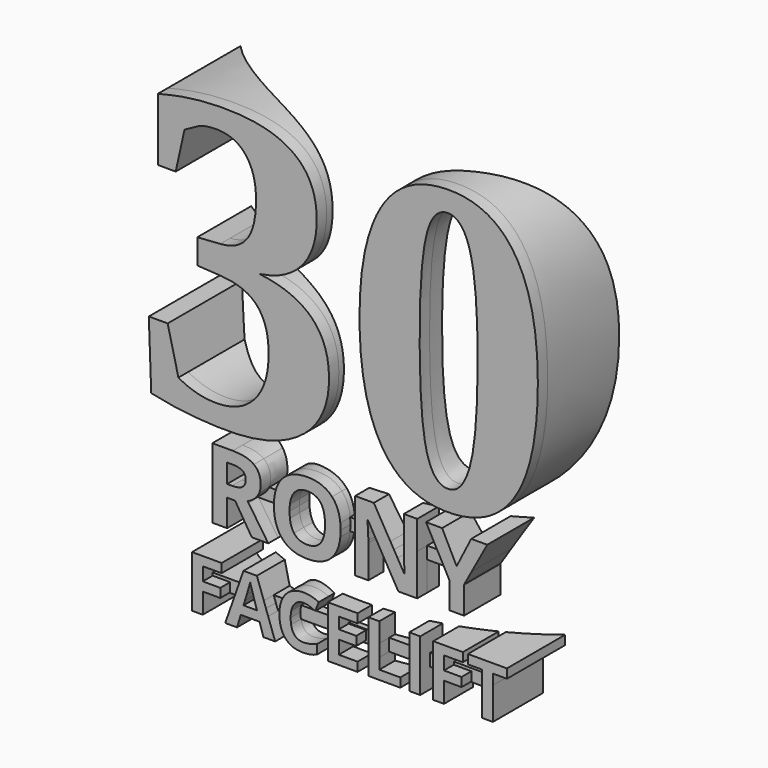
from build123d import *

# Parameters (mm, degrees)
F0_TEXT_SIZE = 68.3343502135
F0_W         = 2.1540381229
F0_H         = 4.7308358373
F0_W_2       = 2.1689621745
F0_H_2       = 4.6338295015
F0_W_3       = 1.7499570325
F0_H_3       = 3.2307460681
F0_W_4       = 1.7793372135
F0_H_4       = 3.1591318768
F0_W_5       = 4.8605836989
F0_H_5       = 1
F0_W_6       = 2.1117005114
F1_DEPTH     = 30
F2_R         = 41.5
F3_DEPTH     = 100
F5_DEPTH     = 2


# Not quite as in the source:
# - Text() gives the source's letters only with a copy of the font that has no kerning and outlines rounded to 1/6400 em; it was checked with that copy


with BuildPart() as f1:
    # F0 (on Front) → F1 (new body)
    with BuildSketch(Plane.XZ):
        with Locations((-35, 14.6143996297)):
            Text('30', F0_TEXT_SIZE, font='Tinos', font_style=FontStyle.BOLD, text_align=(TextAlign.LEFT, TextAlign.BOTTOM))
        with BuildLine():
            Line((-16.2295685047, 4.7308358373), (-22.1137135467, 4.7308358373))
            Line((-22.1137135467, 4.7308358373), (-22.1137135467, 0))
            Line((-22.1137135467, 0), (-19.7034792037, 0))
            Line((-19.7034792037, 0), (-19.7034792037, 4.3603104266))
            Line((-19.7034792037, 4.3603104266), (-18.4224981029, 4.3603104266))
            Line((-18.4224981029, 4.3603104266), (-15.7088080428, 0))
            Line((-15.7088080428, 0), (-13.0349154537, 0))
            add(Edge.make_bspline(
                [(-16.2295685047, 4.7308358373), (-13.7883128068, 1.0866307977), (-13.0349154537, 0)],
                knots=[0.0291905331, 0.0291905331, 0.0291905331, 1, 1, 1], degree=2))
        make_face()
        with Locations((2.1428450841, 2.3654179187)):
            Rectangle(F0_W, F0_H)
        with Locations((10.0625418315, 9.0477505881)):
            Rectangle(F0_W_2, F0_H_2)
        Polygon((17.5671948611, 6.7308358373), (17.521881029, 6.7308358373), (17.5444663969, 6.6859751435), align=None)
        Polygon((17.5671948611, 6.7308358373), (19.994710284, 6.7308358373), (22.5116882576, 11.3646653388), (19.9149032689, 11.3646653388), align=None)
        Polygon((18.9083613052, 4.7308358373), (16.1409885207, 4.7308358373), (16.3480549222, 4.3453863749), (16.3480549222, 0), (18.7408778716, 0), (18.7408778716, 4.4224939751), align=None)
        Polygon((12.5772445362, 11.3646653388), (15.0665732124, 6.7308358373), (17.521881029, 6.7308358373), (15.1889535766, 11.3646653388), align=None)
        with Locations((-24.5407143345, -12.0396394394)):
            Rectangle(F0_W_3, F0_H_3)
        Polygon((-25.4156928507, -5.2651345286), (-25.4156928507, -8.4242664054), (-23.6657358182, -8.4242664054), (-23.6657358182, -6.7231260121), (-20.6065244687, -6.7231260121), (-20.6065244687, -5.2651345286), align=None)
        Polygon((-13.051883354, -10.4242664054), (-18.8849259394, -10.4242664054), (-20.0207571094, -13.6550124735), (-18.1037002973, -13.6550124735), (-17.4958978023, -11.6571601635), (-14.4366864527, -11.6571601635), (-13.8288839577, -13.6550124735), (-11.9118271456, -13.6550124735), align=None)
        with BuildLine():
            add(Edge.make_bspline(
                [(-11.143774011, -8.4242664054), (-11.0275262467, -7.7471500045), (-10.7522281257, -7.1785188181)],
                knots=[0.4222613792, 0.4222613792, 0.4222613792, 1, 1, 1], degree=2))
            Line((-11.143774011, -8.4242664054), (-9.2940985776, -8.4242664054))
            add(Edge.make_bspline(
                [(-8.8471070121, -7.3805075626), (-9.158759552, -7.8074715422), (-9.2940985776, -8.4242664054)],
                knots=[0, 0, 0, 0.5657374533, 0.5657374533, 0.5657374533], degree=2))
            add(Edge.make_bspline(
                [(-7.2917936789, -6.6258041625), (-8.2962286178, -6.6258041625), (-8.8471070121, -7.3805075626)],
                knots=[0, 0, 0, 1, 1, 1], degree=2))
            add(Edge.make_bspline(
                [(-6.35713667, -6.7919858114), (-6.8327283504, -6.6258041625), (-7.2917936789, -6.6258041625)],
                knots=[0, 0, 0, 1, 1, 1], degree=2))
            add(Edge.make_bspline(
                [(-5.4096258318, -7.1821913407), (-5.8815449896, -6.9581674603), (-6.35713667, -6.7919858114)],
                knots=[0, 0, 0, 1, 1, 1], degree=2))
            Line((-5.4096258318, -7.1821913407), (-4.8367123018, -5.7352174251))
            add(Edge.make_bspline(
                [(-7.2917936789, -5.1457775432), (-6.070679905, -5.1457775432), (-4.8367123018, -5.7352174251)],
                knots=[0, 0, 0, 1, 1, 1], degree=2))
            add(Edge.make_bspline(
                [(-9.3832953159, -5.6700301484), (-8.4908723171, -5.1457775432), (-7.2917936789, -5.1457775432)],
                knots=[0, 0, 0, 1, 1, 1], degree=2))
            add(Edge.make_bspline(
                [(-10.7522281257, -7.1785188181), (-10.2757183146, -6.1942827536), (-9.3832953159, -5.6700301484)],
                knots=[0, 0, 0, 1, 1, 1], degree=2))
        make_face()
        with BuildLine():
            Line((-9.3260508973, -10.4242664054), (-11.1714922484, -10.4242664054))
            add(Edge.make_bspline(
                [(-10.2591919628, -12.6597588411), (-10.993148619, -11.8187668393), (-11.1714922484, -10.4242664054)],
                knots=[0, 0, 0, 0.7570106791, 0.7570106791, 0.7570106791], degree=2))
            add(Edge.make_bspline(
                [(-7.4588934585, -13.7706969363), (-9.2896459889, -13.7706969363), (-10.2591919628, -12.6597588411)],
                knots=[0, 0, 0, 1, 1, 1], degree=2))
            add(Edge.make_bspline(
                [(-5.1525492478, -13.3391755274), (-6.1845281064, -13.7706969363), (-7.4588934585, -13.7706969363)],
                knots=[0, 0, 0, 1, 1, 1], degree=2))
            Line((-5.1525492478, -13.3391755274), (-5.1525492478, -11.8481313402))
            add(Edge.make_bspline(
                [(-7.2917936789, -12.2888340557), (-6.4085519868, -12.2888340557), (-5.1525492478, -11.8481313402)],
                knots=[0, 0, 0, 1, 1, 1], degree=2))
            add(Edge.make_bspline(
                [(-9.3260508973, -10.4242664054), (-9.0087452904, -12.2888340557), (-7.2917936789, -12.2888340557)],
                knots=[0.184807542, 0.184807542, 0.184807542, 1, 1, 1], degree=2))
        make_face()
        Polygon((-1.5883660368, -10.4242664054), (-3.3677032504, -10.4242664054), (-3.3677032504, -13.6550124735), (1.4635002675, -13.6550124735), (1.4635002675, -12.1860034221), (-1.5883660368, -12.1860034221), align=None)
        Polygon((-3.3677032504, -5.2651345286), (-3.3677032504, -8.4242664054), (-1.5883660368, -8.4242664054), (-1.5883660368, -6.7231260121), (1.4635002675, -6.7231260121), (1.4635002675, -5.2651345286), align=None)
        Polygon((4.9927945135, -10.4242664054), (3.2134573, -10.4242664054), (3.2134573, -13.6550124735), (8.3953867288, -13.6550124735), (8.3953867288, -12.1860034221), (4.9927945135, -12.1860034221), align=None)
        with Locations((4.1031259067, -6.844700467)):
            Rectangle(F0_W_4, F0_H_4)
        with Locations((10.7430468191, -12.0396394394)):
            Rectangle(F0_W_4, F0_H_3)
        with Locations((10.7430468191, -6.844700467)):
            Rectangle(F0_W_4, F0_H_4)
        with Locations((14.6193944535, -12.0396394394)):
            Rectangle(F0_W_3, F0_H_3)
        Polygon((13.7444159373, -5.2651345286), (13.7444159373, -8.4242664054), (15.4943729697, -8.4242664054), (15.4943729697, -6.7231260121), (18.5535843193, -6.7231260121), (18.5535843193, -5.2651345286), align=None)
        with Locations((22.5428620245, -12.0396394394)):
            Rectangle(F0_W_4, F0_H_3)
        Polygon((21.6531934178, -6.7451611479), (21.6531934178, -8.4242664054), (23.4325306313, -8.4242664054), (23.4325306313, -6.7451611479), (25.709494661, -6.7451611479), (25.709494661, -5.2651345286), (19.3743931268, -5.2651345286), (19.3743931268, -6.7451611479), align=None)
        with BuildLine():
            Line((-22.1137135467, 11.3646653388), (-22.1137135467, 6.7308358373))
            Line((-22.1137135467, 6.7308358373), (-19.7034792037, 6.7308358373))
            Line((-19.7034792037, 6.7308358373), (-19.7034792037, 9.3897158359))
            Line((-19.7034792037, 9.3897158359), (-18.9722006724, 9.3897158359))
            add(Edge.make_bspline(
                [(-17.2522037186, 9.0477063187), (-17.8081246429, 9.3897158359), (-18.9722006724, 9.3897158359)],
                knots=[0, 0, 0, 1, 1, 1], degree=2))
            add(Edge.make_bspline(
                [(-16.6962827943, 7.8973106699), (-16.6962827943, 8.7056968015), (-17.2522037186, 9.0477063187)],
                knots=[0, 0, 0, 1, 1, 1], degree=2))
            add(Edge.make_bspline(
                [(-17.1987400001, 6.7308358373), (-16.6962827943, 7.1128604137), (-16.6962827943, 7.8973106699)],
                knots=[0.0384849815, 0.0384849815, 0.0384849815, 1, 1, 1], degree=2))
            Line((-17.1987400001, 6.7308358373), (-14.5044716431, 6.7308358373))
            add(Edge.make_bspline(
                [(-14.2636623737, 7.9594942185), (-14.2636623737, 7.296785739), (-14.5044716431, 6.7308358373)],
                knots=[0, 0, 0, 0.6611225765, 0.6611225765, 0.6611225765], degree=2))
            add(Edge.make_bspline(
                [(-15.3742605514, 10.5214564201), (-14.2636623737, 9.6782475013), (-14.2636623737, 7.9594942185)],
                knots=[0, 0, 0, 1, 1, 1], degree=2))
            add(Edge.make_bspline(
                [(-18.8030614202, 11.3646653388), (-16.4848587291, 11.3646653388), (-15.3742605514, 10.5214564201)],
                knots=[0, 0, 0, 1, 1, 1], degree=2))
            Line((-18.8030614202, 11.3646653388), (-22.1137135467, 11.3646653388))
        make_face()
        with BuildLine():
            Line((-15.1938905097, 5.7308358373), (-22.1137135467, 5.7308358373))
            Line((-22.1137135467, 5.7308358373), (-22.1137135467, 4.7308358373))
            Line((-22.1137135467, 4.7308358373), (-16.2295685047, 4.7308358373))
            add(Edge.make_bspline(
                [(-16.3779030255, 4.9522978091), (-16.3029727695, 4.8404106729), (-16.2295685047, 4.7308358373)],
                knots=[0, 0, 0, 0.0291905331, 0.0291905331, 0.0291905331], degree=2))
            add(Edge.make_bspline(
                [(-15.1938905097, 5.7308358373), (-15.6745279698, 5.2599163838), (-16.3779030255, 4.9522978091)],
                knots=[0.3052043991, 0.3052043991, 0.3052043991, 1, 1, 1], degree=2))
        make_face()
        with BuildLine():
            add(Edge.make_bspline(
                [(-14.8146086142, 6.1760700452), (-14.9827598304, 5.9376976664), (-15.1938905097, 5.7308358373)],
                knots=[0, 0, 0, 0.3052043991, 0.3052043991, 0.3052043991], degree=2))
            Line((-15.1938905097, 5.7308358373), (-12.1096110315, 5.7308358373))
            add(Edge.make_bspline(
                [(-12.1096110315, 5.7308358373), (-12.1088165409, 6.2536734066), (-12.0602726932, 6.7308358373)],
                knots=[0.0030697124, 0.0030697124, 0.0030697124, 0.1875612566, 0.1875612566, 0.1875612566], degree=2))
            Line((-12.0602726932, 6.7308358373), (-14.5044716431, 6.7308358373))
            add(Edge.make_bspline(
                [(-14.5044716431, 6.7308358373), (-14.6279053717, 6.4407419103), (-14.8146086142, 6.1760700452)],
                knots=[0.6611225765, 0.6611225765, 0.6611225765, 1, 1, 1], degree=2))
        make_face()
        with BuildLine():
            Line((-12.1096110315, 5.7308358373), (-15.1938905097, 5.7308358373))
            add(Edge.make_bspline(
                [(-15.1938905097, 5.7308358373), (-15.6745279698, 5.2599163838), (-16.3779030255, 4.9522978091)],
                knots=[0.3052043991, 0.3052043991, 0.3052043991, 1, 1, 1], degree=2))
            add(Edge.make_bspline(
                [(-16.3779030255, 4.9522978091), (-16.3029727695, 4.8404106729), (-16.2295685047, 4.7308358373)],
                knots=[0, 0, 0, 0.0291905331, 0.0291905331, 0.0291905331], degree=2))
            Line((-16.2295685047, 4.7308358373), (-12.0639311945, 4.7308358373))
            add(Edge.make_bspline(
                [(-12.0639311945, 4.7308358373), (-12.1096242508, 5.2005427099), (-12.1096242508, 5.7134244437)],
                knots=[0.8192842126, 0.8192842126, 0.8192842126, 1, 1, 1], degree=2))
            add(Edge.make_bspline(
                [(-12.1096242508, 5.7134244437), (-12.1096242508, 5.7221364631), (-12.1096110315, 5.7308358373)],
                knots=[0, 0, 0, 0.0030697124, 0.0030697124, 0.0030697124], degree=2))
        make_face()
        with BuildLine():
            Line((1.0658260227, 5.7308358373), (-1.2897322792, 5.7308358373))
            add(Edge.make_bspline(
                [(-1.2897322792, 5.7308358373), (-1.2896867976, 5.7146897348), (-1.2896867976, 5.698500392)],
                knots=[0.9942755567, 0.9942755567, 0.9942755567, 1, 1, 1], degree=2))
            add(Edge.make_bspline(
                [(-1.2896867976, 5.698500392), (-1.2896867976, 5.1937790578), (-1.3344064723, 4.7308358373)],
                knots=[0, 0, 0, 0.1787805659, 0.1787805659, 0.1787805659], degree=2))
            Line((-1.3344064723, 4.7308358373), (1.0658260227, 4.7308358373))
            Line((1.0658260227, 4.7308358373), (1.0658260227, 5.7308358373))
        make_face()
        with BuildLine():
            Line((-9.5289267909, 4.7308358373), (-12.0639311945, 4.7308358373))
            add(Edge.make_bspline(
                [(-10.7104944078, 1.359332372), (-11.8567793996, 2.6013958432), (-12.0639311945, 4.7308358373)],
                knots=[0, 0, 0, 0.8192842126, 0.8192842126, 0.8192842126], degree=2))
            add(Edge.make_bspline(
                [(-6.6996555242, -0.1567025424), (-9.3113645647, -0.1567025424), (-10.7104944078, 1.359332372)],
                knots=[0, 0, 0, 1, 1, 1], degree=2))
            add(Edge.make_bspline(
                [(-2.6888166407, 1.359332372), (-4.0879464838, -0.1567025424), (-6.6996555242, -0.1567025424)],
                knots=[0, 0, 0, 1, 1, 1], degree=2))
            add(Edge.make_bspline(
                [(-1.3344064723, 4.7308358373), (-1.5398240227, 2.6043297065), (-2.6888166407, 1.359332372)],
                knots=[0.1787805659, 0.1787805659, 0.1787805659, 1, 1, 1], degree=2))
            Line((-1.3344064723, 4.7308358373), (-3.8696729528, 4.7308358373))
            add(Edge.make_bspline(
                [(-6.6996555242, 1.8655064575), (-4.2071442024, 1.8655064575), (-3.8696729528, 4.7308358373)],
                knots=[0, 0, 0, 0.8646059311, 0.8646059311, 0.8646059311], degree=2))
            add(Edge.make_bspline(
                [(-8.859912002, 2.8293514605), (-8.1373391674, 1.8655064575), (-6.6996555242, 1.8655064575)],
                knots=[0, 0, 0, 1, 1, 1], degree=2))
            add(Edge.make_bspline(
                [(-9.5289267909, 4.7308358373), (-9.3857627259, 3.530787452), (-8.859912002, 2.8293514605)],
                knots=[0.2722522923, 0.2722522923, 0.2722522923, 1, 1, 1], degree=2))
        make_face()
        with BuildLine():
            add(Edge.make_bspline(
                [(-12.0602726932, 6.7308358373), (-11.8465019058, 8.8320987828), (-10.7067633948, 10.0476177799)],
                knots=[0.1875612566, 0.1875612566, 0.1875612566, 1, 1, 1], degree=2))
            Line((-12.0602726932, 6.7308358373), (-9.5201301427, 6.7308358373))
            add(Edge.make_bspline(
                [(-8.8524499761, 8.5688929946), (-9.3691280927, 7.8840964449), (-9.5201301427, 6.7308358373)],
                knots=[0, 0, 0, 0.7077444443, 0.7077444443, 0.7077444443], degree=2))
            add(Edge.make_bspline(
                [(-6.6847314726, 9.5364690105), (-8.1224151158, 9.5364690105), (-8.8524499761, 8.5688929946)],
                knots=[0, 0, 0, 1, 1, 1], degree=2))
            add(Edge.make_bspline(
                [(-3.8771261804, 6.7308358373), (-4.2326802689, 9.5364690105), (-6.6847314726, 9.5364690105)],
                knots=[0.1450027177, 0.1450027177, 0.1450027177, 1, 1, 1], degree=2))
            Line((-3.8771261804, 6.7308358373), (-1.3403341394, 6.7308358373))
            add(Edge.make_bspline(
                [(-2.6776236019, 10.0351810702), (-1.5548194244, 8.8147854901), (-1.3403341394, 6.7308358373)],
                knots=[0, 0, 0, 0.8089735599, 0.8089735599, 0.8089735599], degree=2))
            add(Edge.make_bspline(
                [(-6.6847314726, 11.5437539588), (-4.0655604063, 11.5437539588), (-2.6776236019, 10.0351810702)],
                knots=[0, 0, 0, 1, 1, 1], degree=2))
            add(Edge.make_bspline(
                [(-10.7067633948, 10.0476177799), (-9.3039025388, 11.5437539588), (-6.6847314726, 11.5437539588)],
                knots=[0, 0, 0, 1, 1, 1], degree=2))
        make_face()
        with BuildLine():
            add(Edge.make_bspline(
                [(-1.3403341394, 6.7308358373), (-1.2912045343, 6.2534901601), (-1.2897322792, 5.7308358373)],
                knots=[0.8089735599, 0.8089735599, 0.8089735599, 0.9942755567, 0.9942755567, 0.9942755567], degree=2))
            Line((-1.2897322792, 5.7308358373), (1.0658260227, 5.7308358373))
            Line((1.0658260227, 5.7308358373), (1.0658260227, 6.7308358373))
            Line((1.0658260227, 6.7308358373), (-1.3403341394, 6.7308358373))
        make_face()
        with BuildLine():
            Line((7.9515056655, 4.7308358373), (5.3637792793, 4.7308358373))
            Line((5.3637792793, 4.7308358373), (8.0851049866, 0))
            Line((8.0851049866, 0), (11.1470229188, 0))
            Line((11.1470229188, 0), (11.1470229188, 4.7308358373))
            Line((11.1470229188, 4.7308358373), (9.0077790091, 4.7308358373))
            add(Edge.make_bspline(
                [(9.0949658156, 2.8529812089), (9.0370032236, 3.951803964), (9.0077790091, 4.7308358373)],
                knots=[0, 0, 0, 0.4958090471, 0.4958090471, 0.4958090471], degree=2))
            Line((9.0949658156, 2.8529812089), (9.0402442928, 2.8529812089))
            Line((9.0402442928, 2.8529812089), (7.9515056655, 4.7308358373))
        make_face()
        with BuildLine():
            Line((1.0658260227, 11.3646653388), (1.0658260227, 6.7308358373))
            Line((1.0658260227, 6.7308358373), (3.1786052124, 6.7308358373))
            add(Edge.make_bspline(
                [(3.070623629, 8.596253756), (3.1413943775, 7.5169998403), (3.1786052124, 6.7308358373)],
                knots=[0, 0, 0, 0.474206001, 0.474206001, 0.474206001], degree=2))
            Line((3.070623629, 8.596253756), (3.1402692034, 8.596253756))
            Line((3.1402692034, 8.596253756), (4.2133163163, 6.7308358373))
            Line((4.2133163163, 6.7308358373), (6.7919498502, 6.7308358373))
            Line((6.7919498502, 6.7308358373), (4.1053578774, 11.3646653388))
            Line((4.1053578774, 11.3646653388), (1.0658260227, 11.3646653388))
        make_face()
        Polygon((11.1470229188, 6.7308358373), (11.1470229188, 5.7308358373), (15.6037808666, 5.7308358373), (15.0665732124, 6.7308358373), align=None)
        Polygon((15.6037808666, 5.7308358373), (11.1470229188, 5.7308358373), (11.1470229188, 4.7308358373), (16.1409885207, 4.7308358373), align=None)
        Polygon((19.4515357946, 5.7308358373), (15.6037808666, 5.7308358373), (16.1409885207, 4.7308358373), (18.9083613052, 4.7308358373), align=None)
        Polygon((-20.8195307811, -9.4242664054), (-25.4156928507, -9.4242664054), (-25.4156928507, -10.4242664054), (-23.6657358182, -10.4242664054), (-23.6657358182, -10.3387245399), (-20.8195307811, -10.3387245399), align=None)
        Polygon((-25.4156928507, -8.4242664054), (-25.4156928507, -9.4242664054), (-20.8195307811, -9.4242664054), (-20.8195307811, -8.8862418403), (-23.6657358182, -8.8862418403), (-23.6657358182, -8.4242664054), align=None)
        Polygon((-20.8195307811, -8.8862418403), (-20.8195307811, -9.4242664054), (-18.5333566282, -9.4242664054), (-18.1817873169, -8.4242664054), (-23.6657358182, -8.4242664054), (-23.6657358182, -8.8862418403), align=None)
        Polygon((-18.5333566282, -9.4242664054), (-20.8195307811, -9.4242664054), (-20.8195307811, -10.3387245399), (-23.6657358182, -10.3387245399), (-23.6657358182, -10.4242664054), (-18.8849259394, -10.4242664054), align=None)
        with BuildLine():
            Line((-17.0588676095, -5.2302455636), (-18.1817873169, -8.4242664054))
            Line((-18.1817873169, -8.4242664054), (-16.5147517741, -8.4242664054))
            add(Edge.make_bspline(
                [(-15.9644558662, -6.5339910968), (-16.0883411528, -7.0150990059), (-16.5147517741, -8.4242664054)],
                knots=[0, 0, 0, 0.6550101359, 0.6550101359, 0.6550101359], degree=2))
            add(Edge.make_bspline(
                [(-15.8120461771, -7.0958870589), (-15.9185493333, -6.739652364), (-15.9644558662, -6.5339910968)],
                knots=[0, 0, 0, 1, 1, 1], degree=2))
            add(Edge.make_bspline(
                [(-15.403025702, -8.4242664054), (-15.7465925318, -7.3148182173), (-15.8120461771, -7.0958870589)],
                knots=[0.3854299947, 0.3854299947, 0.3854299947, 1, 1, 1], degree=2))
            Line((-15.403025702, -8.4242664054), (-13.7576374953, -8.4242664054))
            Line((-13.7576374953, -8.4242664054), (-14.8847342134, -5.2302455636))
            Line((-14.8847342134, -5.2302455636), (-17.0588676095, -5.2302455636))
        make_face()
        with BuildLine():
            Line((-13.7576374953, -8.4242664054), (-13.4047604246, -9.4242664054))
            Line((-13.4047604246, -9.4242664054), (-11.2285788068, -9.4242664054))
            add(Edge.make_bspline(
                [(-11.2285788068, -9.4242664054), (-11.22506094, -8.8977440085), (-11.143774011, -8.4242664054)],
                knots=[0.01827427, 0.01827427, 0.01827427, 0.4222613792, 0.4222613792, 0.4222613792], degree=2))
            Line((-11.143774011, -8.4242664054), (-13.7576374953, -8.4242664054))
        make_face()
        with BuildLine():
            Line((-13.4047604246, -9.4242664054), (-13.051883354, -10.4242664054))
            Line((-13.051883354, -10.4242664054), (-11.1714922484, -10.4242664054))
            add(Edge.make_bspline(
                [(-11.1714922484, -10.4242664054), (-11.2287379367, -9.9766522268), (-11.2287379367, -9.4720091996)],
                knots=[0.7570106791, 0.7570106791, 0.7570106791, 1, 1, 1], degree=2))
            add(Edge.make_bspline(
                [(-11.2287379367, -9.4720091996), (-11.2287379367, -9.4480835327), (-11.2285788068, -9.4242664054)],
                knots=[0, 0, 0, 0.01827427, 0.01827427, 0.01827427], degree=2))
            Line((-11.2285788068, -9.4242664054), (-13.4047604246, -9.4242664054))
        make_face()
        with BuildLine():
            add(Edge.make_bspline(
                [(-9.2940985776, -8.4242664054), (-9.39274542, -8.8738400989), (-9.3977211048, -9.4242664054)],
                knots=[0.5657374533, 0.5657374533, 0.5657374533, 0.9780960697, 0.9780960697, 0.9780960697], degree=2))
            Line((-9.3977211048, -9.4242664054), (-3.3677032504, -9.4242664054))
            Line((-3.3677032504, -9.4242664054), (-3.3677032504, -8.4242664054))
            Line((-3.3677032504, -8.4242664054), (-9.2940985776, -8.4242664054))
        make_face()
        with BuildLine():
            add(Edge.make_bspline(
                [(-9.3979854064, -9.4830267675), (-9.3979854064, -10.0015611156), (-9.3260508973, -10.4242664054)],
                knots=[0, 0, 0, 0.184807542, 0.184807542, 0.184807542], degree=2))
            Line((-9.3260508973, -10.4242664054), (-3.3677032504, -10.4242664054))
            Line((-3.3677032504, -10.4242664054), (-3.3677032504, -9.4242664054))
            Line((-3.3677032504, -9.4242664054), (-9.3977211048, -9.4242664054))
            add(Edge.make_bspline(
                [(-9.3977211048, -9.4242664054), (-9.3979854064, -9.4535043041), (-9.3979854064, -9.4830267675)],
                knots=[0.9780960697, 0.9780960697, 0.9780960697, 1, 1, 1], degree=2))
        make_face()
        Polygon((1.2523302163, -8.5648961103), (1.2523302163, -9.4242664054), (3.2134573, -9.4242664054), (3.2134573, -8.4242664054), (-1.5883660368, -8.4242664054), (-1.5883660368, -8.5648961103), align=None)
        Polygon((-1.5883660368, -10.0228875939), (-1.5883660368, -10.4242664054), (3.2134573, -10.4242664054), (3.2134573, -9.4242664054), (1.2523302163, -9.4242664054), (1.2523302163, -10.0228875939), align=None)
        with Locations((7.4230863629, -8.9242664054)):
            Rectangle(F0_W_5, F0_H_5)
        with Locations((7.4230863629, -9.9242664054)):
            Rectangle(F0_W_5, F0_H_5)
        with Locations((12.6885656816, -8.9242664054)):
            Rectangle(F0_W_6, F0_H_5)
        with Locations((12.6885656816, -9.9242664054)):
            Rectangle(F0_W_6, F0_H_5)
        Polygon((18.3405780069, -8.8862418403), (18.3405780069, -9.4242664054), (21.6531934178, -9.4242664054), (21.6531934178, -8.4242664054), (15.4943729697, -8.4242664054), (15.4943729697, -8.8862418403), align=None)
        Polygon((15.4943729697, -10.3387245399), (15.4943729697, -10.4242664054), (21.6531934178, -10.4242664054), (21.6531934178, -9.4242664054), (18.3405780069, -9.4242664054), (18.3405780069, -10.3387245399), align=None)
        with Locations((22.5428620245, -9.9242664054)):
            Rectangle(F0_W_4, F0_H_5)
        with Locations((22.5428620245, -8.9242664054)):
            Rectangle(F0_W_4, F0_H_5)
        with BuildLine():
            Line((-22.1137135467, 6.7308358373), (-22.1137135467, 5.7308358373))
            Line((-22.1137135467, 5.7308358373), (-15.1938905097, 5.7308358373))
            add(Edge.make_bspline(
                [(-14.8146086142, 6.1760700452), (-14.9827598304, 5.9376976664), (-15.1938905097, 5.7308358373)],
                knots=[0, 0, 0, 0.3052043991, 0.3052043991, 0.3052043991], degree=2))
            add(Edge.make_bspline(
                [(-14.5044716431, 6.7308358373), (-14.6279053717, 6.4407419103), (-14.8146086142, 6.1760700452)],
                knots=[0.6611225765, 0.6611225765, 0.6611225765, 1, 1, 1], degree=2))
            Line((-14.5044716431, 6.7308358373), (-17.1987400001, 6.7308358373))
            add(Edge.make_bspline(
                [(-17.2397670089, 6.7008991952), (-17.2188510289, 6.7155451674), (-17.1987400001, 6.7308358373)],
                knots=[0, 0, 0, 0.0384849815, 0.0384849815, 0.0384849815], degree=2))
            add(Edge.make_bspline(
                [(-18.9274285174, 6.3203358779), (-17.7832512235, 6.3203358779), (-17.2397670089, 6.7008991952)],
                knots=[0, 0, 0, 1, 1, 1], degree=2))
            Line((-18.9274285174, 6.3203358779), (-19.7034792037, 6.3203358779))
            Line((-19.7034792037, 6.3203358779), (-19.7034792037, 6.7308358373))
            Line((-19.7034792037, 6.7308358373), (-22.1137135467, 6.7308358373))
        make_face()
        with BuildLine():
            Line((-1.2897322792, 5.7308358373), (-3.8168773207, 5.7308358373))
            add(Edge.make_bspline(
                [(-3.816826212, 5.698500392), (-3.816826212, 5.7147023128), (-3.8168773207, 5.7308358373)],
                knots=[0, 0, 0, 0.0042214834, 0.0042214834, 0.0042214834], degree=2))
            add(Edge.make_bspline(
                [(-3.8696729528, 4.7308358373), (-3.816826212, 5.1795357472), (-3.816826212, 5.698500392)],
                knots=[0.8646059311, 0.8646059311, 0.8646059311, 1, 1, 1], degree=2))
            Line((-3.8696729528, 4.7308358373), (-1.3344064723, 4.7308358373))
            add(Edge.make_bspline(
                [(-1.2896867976, 5.698500392), (-1.2896867976, 5.1937790578), (-1.3344064723, 4.7308358373)],
                knots=[0, 0, 0, 0.1787805659, 0.1787805659, 0.1787805659], degree=2))
            add(Edge.make_bspline(
                [(-1.2897322792, 5.7308358373), (-1.2896867976, 5.7146897348), (-1.2896867976, 5.698500392)],
                knots=[0.9942755567, 0.9942755567, 0.9942755567, 1, 1, 1], degree=2))
        make_face()
        with BuildLine():
            Line((-9.5824319108, 5.7308358373), (-12.1096110315, 5.7308358373))
            add(Edge.make_bspline(
                [(-12.1096242508, 5.7134244437), (-12.1096242508, 5.7221364631), (-12.1096110315, 5.7308358373)],
                knots=[0, 0, 0, 0.0030697124, 0.0030697124, 0.0030697124], degree=2))
            add(Edge.make_bspline(
                [(-12.0639311945, 4.7308358373), (-12.1096242508, 5.2005427099), (-12.1096242508, 5.7134244437)],
                knots=[0.8192842126, 0.8192842126, 0.8192842126, 1, 1, 1], degree=2))
            Line((-12.0639311945, 4.7308358373), (-9.5289267909, 4.7308358373))
            add(Edge.make_bspline(
                [(-9.5824848365, 5.698500392), (-9.5824848365, 5.1797770299), (-9.5289267909, 4.7308358373)],
                knots=[0, 0, 0, 0.2722522923, 0.2722522923, 0.2722522923], degree=2))
            add(Edge.make_bspline(
                [(-9.5824319108, 5.7308358373), (-9.5824848365, 5.714702016), (-9.5824848365, 5.698500392)],
                knots=[0.9914854516, 0.9914854516, 0.9914854516, 1, 1, 1], degree=2))
        make_face()
        with BuildLine():
            add(Edge.make_bspline(
                [(-12.1096110315, 5.7308358373), (-12.1088165409, 6.2536734066), (-12.0602726932, 6.7308358373)],
                knots=[0.0030697124, 0.0030697124, 0.0030697124, 0.1875612566, 0.1875612566, 0.1875612566], degree=2))
            Line((-12.1096110315, 5.7308358373), (-9.5824319108, 5.7308358373))
            add(Edge.make_bspline(
                [(-9.5201301427, 6.7308358373), (-9.5806682002, 6.2684834598), (-9.5824319108, 5.7308358373)],
                knots=[0.7077444443, 0.7077444443, 0.7077444443, 0.9914854516, 0.9914854516, 0.9914854516], degree=2))
            Line((-9.5201301427, 6.7308358373), (-12.0602726932, 6.7308358373))
        make_face()
        with BuildLine():
            add(Edge.make_bspline(
                [(-3.8168773207, 5.7308358373), (-3.8185817329, 6.2688688704), (-3.8771261804, 6.7308358373)],
                knots=[0.0042214834, 0.0042214834, 0.0042214834, 0.1450027177, 0.1450027177, 0.1450027177], degree=2))
            Line((-3.8168773207, 5.7308358373), (-1.2897322792, 5.7308358373))
            add(Edge.make_bspline(
                [(-1.3403341394, 6.7308358373), (-1.2912045343, 6.2534901601), (-1.2897322792, 5.7308358373)],
                knots=[0.8089735599, 0.8089735599, 0.8089735599, 0.9942755567, 0.9942755567, 0.9942755567], degree=2))
            Line((-1.3403341394, 6.7308358373), (-3.8771261804, 6.7308358373))
        make_face()
        Polygon((7.3717277579, 5.7308358373), (4.7885477978, 5.7308358373), (5.3637792793, 4.7308358373), (7.9515056655, 4.7308358373), align=None)
        Polygon((4.2133163163, 6.7308358373), (4.7885477978, 5.7308358373), (7.3717277579, 5.7308358373), (6.7919498502, 6.7308358373), align=None)
        with BuildLine():
            Line((1.0658260227, 6.7308358373), (1.0658260227, 5.7308358373))
            Line((1.0658260227, 5.7308358373), (3.2152338451, 5.7308358373))
            add(Edge.make_bspline(
                [(3.1786052124, 6.7308358373), (3.2060423781, 6.1511629533), (3.2152338451, 5.7308358373)],
                knots=[0.474206001, 0.474206001, 0.474206001, 0.8238586933, 0.8238586933, 0.8238586933], degree=2))
            Line((3.1786052124, 6.7308358373), (1.0658260227, 6.7308358373))
        make_face()
        with BuildLine():
            Line((3.2152338451, 5.7308358373), (1.0658260227, 5.7308358373))
            Line((1.0658260227, 5.7308358373), (1.0658260227, 4.7308358373))
            Line((1.0658260227, 4.7308358373), (3.2198641456, 4.7308358373))
            Line((3.2198641456, 4.7308358373), (3.2198641456, 5.347785178))
            add(Edge.make_bspline(
                [(3.2152338451, 5.7308358373), (3.2198641456, 5.5190915291), (3.2198641456, 5.347785178)],
                knots=[0.8238586933, 0.8238586933, 0.8238586933, 1, 1, 1], degree=2))
        make_face()
        with BuildLine():
            Line((11.1470229188, 5.7308358373), (8.9799494697, 5.7308358373))
            add(Edge.make_bspline(
                [(9.0077790091, 4.7308358373), (8.9855527162, 5.3233236381), (8.9799494697, 5.7308358373)],
                knots=[0.4958090471, 0.4958090471, 0.4958090471, 0.8728935053, 0.8728935053, 0.8728935053], degree=2))
            Line((9.0077790091, 4.7308358373), (11.1470229188, 4.7308358373))
            Line((11.1470229188, 4.7308358373), (11.1470229188, 5.7308358373))
        make_face()
        with BuildLine():
            add(Edge.make_bspline(
                [(8.9799494697, 5.7308358373), (8.9780607443, 5.8681988234), (8.9780607443, 5.9845447155)],
                knots=[0.8728935053, 0.8728935053, 0.8728935053, 1, 1, 1], degree=2))
            Line((8.9799494697, 5.7308358373), (11.1470229188, 5.7308358373))
            Line((11.1470229188, 5.7308358373), (11.1470229188, 6.7308358373))
            Line((11.1470229188, 6.7308358373), (8.9780607443, 6.7308358373))
            Line((8.9780607443, 6.7308358373), (8.9780607443, 5.9845447155))
        make_face()
        with BuildLine():
            Line((-18.1817873169, -8.4242664054), (-18.5333566282, -9.4242664054))
            Line((-18.5333566282, -9.4242664054), (-16.8195837173, -9.4242664054))
            add(Edge.make_bspline(
                [(-16.5147517741, -8.4242664054), (-16.6515904094, -8.8764796811), (-16.8195837173, -9.4242664054)],
                knots=[0.6550101359, 0.6550101359, 0.6550101359, 0.865208214, 0.865208214, 0.865208214], degree=2))
            Line((-16.5147517741, -8.4242664054), (-18.1817873169, -8.4242664054))
        make_face()
        with BuildLine():
            add(Edge.make_bspline(
                [(-15.0929961456, -9.4242664054), (-15.269131016, -8.8566399756), (-15.403025702, -8.4242664054)],
                knots=[0.1459200922, 0.1459200922, 0.1459200922, 0.3854299947, 0.3854299947, 0.3854299947], degree=2))
            Line((-15.0929961456, -9.4242664054), (-13.4047604246, -9.4242664054))
            Line((-13.4047604246, -9.4242664054), (-13.7576374953, -8.4242664054))
            Line((-13.7576374953, -8.4242664054), (-15.403025702, -8.4242664054))
        make_face()
        with BuildLine():
            add(Edge.make_bspline(
                [(-11.2285788068, -9.4242664054), (-11.22506094, -8.8977440085), (-11.143774011, -8.4242664054)],
                knots=[0.01827427, 0.01827427, 0.01827427, 0.4222613792, 0.4222613792, 0.4222613792], degree=2))
            Line((-11.2285788068, -9.4242664054), (-9.3977211048, -9.4242664054))
            add(Edge.make_bspline(
                [(-9.2940985776, -8.4242664054), (-9.39274542, -8.8738400989), (-9.3977211048, -9.4242664054)],
                knots=[0.5657374533, 0.5657374533, 0.5657374533, 0.9780960697, 0.9780960697, 0.9780960697], degree=2))
            Line((-9.2940985776, -8.4242664054), (-11.143774011, -8.4242664054))
        make_face()
        with BuildLine():
            add(Edge.make_bspline(
                [(-11.1714922484, -10.4242664054), (-11.2287379367, -9.9766522268), (-11.2287379367, -9.4720091996)],
                knots=[0.7570106791, 0.7570106791, 0.7570106791, 1, 1, 1], degree=2))
            Line((-11.1714922484, -10.4242664054), (-9.3260508973, -10.4242664054))
            add(Edge.make_bspline(
                [(-9.3979854064, -9.4830267675), (-9.3979854064, -10.0015611156), (-9.3260508973, -10.4242664054)],
                knots=[0, 0, 0, 0.184807542, 0.184807542, 0.184807542], degree=2))
            add(Edge.make_bspline(
                [(-9.3977211048, -9.4242664054), (-9.3979854064, -9.4535043041), (-9.3979854064, -9.4830267675)],
                knots=[0.9780960697, 0.9780960697, 0.9780960697, 1, 1, 1], degree=2))
            Line((-9.3977211048, -9.4242664054), (-11.2285788068, -9.4242664054))
            add(Edge.make_bspline(
                [(-11.2287379367, -9.4720091996), (-11.2287379367, -9.4480835327), (-11.2285788068, -9.4242664054)],
                knots=[0, 0, 0, 0.01827427, 0.01827427, 0.01827427], degree=2))
        make_face()
        Polygon((-3.3677032504, -9.4242664054), (-3.3677032504, -10.4242664054), (-1.5883660368, -10.4242664054), (-1.5883660368, -10.0228875939), (1.2523302163, -10.0228875939), (1.2523302163, -9.4242664054), align=None)
        Polygon((-3.3677032504, -8.4242664054), (-3.3677032504, -9.4242664054), (1.2523302163, -9.4242664054), (1.2523302163, -8.5648961103), (-1.5883660368, -8.5648961103), (-1.5883660368, -8.4242664054), align=None)
        with Locations((4.1031259067, -9.9242664054)):
            Rectangle(F0_W_4, F0_H_5)
        with Locations((4.1031259067, -8.9242664054)):
            Rectangle(F0_W_4, F0_H_5)
        with Locations((10.7430468191, -9.9242664054)):
            Rectangle(F0_W_4, F0_H_5)
        with Locations((10.7430468191, -8.9242664054)):
            Rectangle(F0_W_4, F0_H_5)
        Polygon((13.7444159373, -9.4242664054), (13.7444159373, -10.4242664054), (15.4943729697, -10.4242664054), (15.4943729697, -10.3387245399), (18.3405780069, -10.3387245399), (18.3405780069, -9.4242664054), align=None)
        Polygon((13.7444159373, -8.4242664054), (13.7444159373, -9.4242664054), (18.3405780069, -9.4242664054), (18.3405780069, -8.8862418403), (15.4943729697, -8.8862418403), (15.4943729697, -8.4242664054), align=None)
        Polygon((15.0665732124, 6.7308358373), (15.6037808666, 5.7308358373), (19.4515357946, 5.7308358373), (19.994710284, 6.7308358373), (17.5671948611, 6.7308358373), (17.5444663969, 6.6859751435), (17.521881029, 6.7308358373), align=None)
        with BuildLine():
            Line((-16.8195837173, -9.4242664054), (-18.5333566282, -9.4242664054))
            Line((-18.5333566282, -9.4242664054), (-18.8849259394, -10.4242664054))
            Line((-18.8849259394, -10.4242664054), (-13.051883354, -10.4242664054))
            Line((-13.051883354, -10.4242664054), (-13.4047604246, -9.4242664054))
            Line((-13.4047604246, -9.4242664054), (-15.0929961456, -9.4242664054))
            add(Edge.make_bspline(
                [(-14.8626990776, -10.1661159764), (-14.9856869435, -9.7700896892), (-15.0929961456, -9.4242664054)],
                knots=[0, 0, 0, 0.1459200922, 0.1459200922, 0.1459200922], degree=2))
            Line((-14.8626990776, -10.1661159764), (-17.0478500416, -10.1661159764))
            add(Edge.make_bspline(
                [(-16.8195837173, -9.4242664054), (-16.9273112388, -9.7755405538), (-17.0478500416, -10.1661159764)],
                knots=[0.865208214, 0.865208214, 0.865208214, 1, 1, 1], degree=2))
        make_face()
    extrude(amount=-F1_DEPTH)

    # F0 (on Front) → F5 (join)
    with BuildSketch(Plane.XZ):
        with Locations((-35, 14.6143996297)):
            Text('30', F0_TEXT_SIZE, font='Tinos', font_style=FontStyle.BOLD, text_align=(TextAlign.LEFT, TextAlign.BOTTOM))
        with BuildLine():
            Line((-16.2295685047, 4.7308358373), (-22.1137135467, 4.7308358373))
            Line((-22.1137135467, 4.7308358373), (-22.1137135467, 0))
            Line((-22.1137135467, 0), (-19.7034792037, 0))
            Line((-19.7034792037, 0), (-19.7034792037, 4.3603104266))
            Line((-19.7034792037, 4.3603104266), (-18.4224981029, 4.3603104266))
            Line((-18.4224981029, 4.3603104266), (-15.7088080428, 0))
            Line((-15.7088080428, 0), (-13.0349154537, 0))
            add(Edge.make_bspline(
                [(-16.2295685047, 4.7308358373), (-13.7883128068, 1.0866307977), (-13.0349154537, 0)],
                knots=[0.0291905331, 0.0291905331, 0.0291905331, 1, 1, 1], degree=2))
        make_face()
        with BuildLine():
            Line((-22.1137135467, 6.7308358373), (-22.1137135467, 5.7308358373))
            Line((-22.1137135467, 5.7308358373), (-15.1938905097, 5.7308358373))
            add(Edge.make_bspline(
                [(-14.8146086142, 6.1760700452), (-14.9827598304, 5.9376976664), (-15.1938905097, 5.7308358373)],
                knots=[0, 0, 0, 0.3052043991, 0.3052043991, 0.3052043991], degree=2))
            add(Edge.make_bspline(
                [(-14.5044716431, 6.7308358373), (-14.6279053717, 6.4407419103), (-14.8146086142, 6.1760700452)],
                knots=[0.6611225765, 0.6611225765, 0.6611225765, 1, 1, 1], degree=2))
            Line((-14.5044716431, 6.7308358373), (-17.1987400001, 6.7308358373))
            add(Edge.make_bspline(
                [(-17.2397670089, 6.7008991952), (-17.2188510289, 6.7155451674), (-17.1987400001, 6.7308358373)],
                knots=[0, 0, 0, 0.0384849815, 0.0384849815, 0.0384849815], degree=2))
            add(Edge.make_bspline(
                [(-18.9274285174, 6.3203358779), (-17.7832512235, 6.3203358779), (-17.2397670089, 6.7008991952)],
                knots=[0, 0, 0, 1, 1, 1], degree=2))
            Line((-18.9274285174, 6.3203358779), (-19.7034792037, 6.3203358779))
            Line((-19.7034792037, 6.3203358779), (-19.7034792037, 6.7308358373))
            Line((-19.7034792037, 6.7308358373), (-22.1137135467, 6.7308358373))
        make_face()
        with BuildLine():
            Line((-15.1938905097, 5.7308358373), (-22.1137135467, 5.7308358373))
            Line((-22.1137135467, 5.7308358373), (-22.1137135467, 4.7308358373))
            Line((-22.1137135467, 4.7308358373), (-16.2295685047, 4.7308358373))
            add(Edge.make_bspline(
                [(-16.3779030255, 4.9522978091), (-16.3029727695, 4.8404106729), (-16.2295685047, 4.7308358373)],
                knots=[0, 0, 0, 0.0291905331, 0.0291905331, 0.0291905331], degree=2))
            add(Edge.make_bspline(
                [(-15.1938905097, 5.7308358373), (-15.6745279698, 5.2599163838), (-16.3779030255, 4.9522978091)],
                knots=[0.3052043991, 0.3052043991, 0.3052043991, 1, 1, 1], degree=2))
        make_face()
        with BuildLine():
            Line((-22.1137135467, 11.3646653388), (-22.1137135467, 6.7308358373))
            Line((-22.1137135467, 6.7308358373), (-19.7034792037, 6.7308358373))
            Line((-19.7034792037, 6.7308358373), (-19.7034792037, 9.3897158359))
            Line((-19.7034792037, 9.3897158359), (-18.9722006724, 9.3897158359))
            add(Edge.make_bspline(
                [(-17.2522037186, 9.0477063187), (-17.8081246429, 9.3897158359), (-18.9722006724, 9.3897158359)],
                knots=[0, 0, 0, 1, 1, 1], degree=2))
            add(Edge.make_bspline(
                [(-16.6962827943, 7.8973106699), (-16.6962827943, 8.7056968015), (-17.2522037186, 9.0477063187)],
                knots=[0, 0, 0, 1, 1, 1], degree=2))
            add(Edge.make_bspline(
                [(-17.1987400001, 6.7308358373), (-16.6962827943, 7.1128604137), (-16.6962827943, 7.8973106699)],
                knots=[0.0384849815, 0.0384849815, 0.0384849815, 1, 1, 1], degree=2))
            Line((-17.1987400001, 6.7308358373), (-14.5044716431, 6.7308358373))
            add(Edge.make_bspline(
                [(-14.2636623737, 7.9594942185), (-14.2636623737, 7.296785739), (-14.5044716431, 6.7308358373)],
                knots=[0, 0, 0, 0.6611225765, 0.6611225765, 0.6611225765], degree=2))
            add(Edge.make_bspline(
                [(-15.3742605514, 10.5214564201), (-14.2636623737, 9.6782475013), (-14.2636623737, 7.9594942185)],
                knots=[0, 0, 0, 1, 1, 1], degree=2))
            add(Edge.make_bspline(
                [(-18.8030614202, 11.3646653388), (-16.4848587291, 11.3646653388), (-15.3742605514, 10.5214564201)],
                knots=[0, 0, 0, 1, 1, 1], degree=2))
            Line((-18.8030614202, 11.3646653388), (-22.1137135467, 11.3646653388))
        make_face()
        with BuildLine():
            add(Edge.make_bspline(
                [(-12.0602726932, 6.7308358373), (-11.8465019058, 8.8320987828), (-10.7067633948, 10.0476177799)],
                knots=[0.1875612566, 0.1875612566, 0.1875612566, 1, 1, 1], degree=2))
            Line((-12.0602726932, 6.7308358373), (-9.5201301427, 6.7308358373))
            add(Edge.make_bspline(
                [(-8.8524499761, 8.5688929946), (-9.3691280927, 7.8840964449), (-9.5201301427, 6.7308358373)],
                knots=[0, 0, 0, 0.7077444443, 0.7077444443, 0.7077444443], degree=2))
            add(Edge.make_bspline(
                [(-6.6847314726, 9.5364690105), (-8.1224151158, 9.5364690105), (-8.8524499761, 8.5688929946)],
                knots=[0, 0, 0, 1, 1, 1], degree=2))
            add(Edge.make_bspline(
                [(-3.8771261804, 6.7308358373), (-4.2326802689, 9.5364690105), (-6.6847314726, 9.5364690105)],
                knots=[0.1450027177, 0.1450027177, 0.1450027177, 1, 1, 1], degree=2))
            Line((-3.8771261804, 6.7308358373), (-1.3403341394, 6.7308358373))
            add(Edge.make_bspline(
                [(-2.6776236019, 10.0351810702), (-1.5548194244, 8.8147854901), (-1.3403341394, 6.7308358373)],
                knots=[0, 0, 0, 0.8089735599, 0.8089735599, 0.8089735599], degree=2))
            add(Edge.make_bspline(
                [(-6.6847314726, 11.5437539588), (-4.0655604063, 11.5437539588), (-2.6776236019, 10.0351810702)],
                knots=[0, 0, 0, 1, 1, 1], degree=2))
            add(Edge.make_bspline(
                [(-10.7067633948, 10.0476177799), (-9.3039025388, 11.5437539588), (-6.6847314726, 11.5437539588)],
                knots=[0, 0, 0, 1, 1, 1], degree=2))
        make_face()
        with BuildLine():
            add(Edge.make_bspline(
                [(-12.1096110315, 5.7308358373), (-12.1088165409, 6.2536734066), (-12.0602726932, 6.7308358373)],
                knots=[0.0030697124, 0.0030697124, 0.0030697124, 0.1875612566, 0.1875612566, 0.1875612566], degree=2))
            Line((-12.1096110315, 5.7308358373), (-9.5824319108, 5.7308358373))
            add(Edge.make_bspline(
                [(-9.5201301427, 6.7308358373), (-9.5806682002, 6.2684834598), (-9.5824319108, 5.7308358373)],
                knots=[0.7077444443, 0.7077444443, 0.7077444443, 0.9914854516, 0.9914854516, 0.9914854516], degree=2))
            Line((-9.5201301427, 6.7308358373), (-12.0602726932, 6.7308358373))
        make_face()
        with BuildLine():
            Line((-9.5824319108, 5.7308358373), (-12.1096110315, 5.7308358373))
            add(Edge.make_bspline(
                [(-12.1096242508, 5.7134244437), (-12.1096242508, 5.7221364631), (-12.1096110315, 5.7308358373)],
                knots=[0, 0, 0, 0.0030697124, 0.0030697124, 0.0030697124], degree=2))
            add(Edge.make_bspline(
                [(-12.0639311945, 4.7308358373), (-12.1096242508, 5.2005427099), (-12.1096242508, 5.7134244437)],
                knots=[0.8192842126, 0.8192842126, 0.8192842126, 1, 1, 1], degree=2))
            Line((-12.0639311945, 4.7308358373), (-9.5289267909, 4.7308358373))
            add(Edge.make_bspline(
                [(-9.5824848365, 5.698500392), (-9.5824848365, 5.1797770299), (-9.5289267909, 4.7308358373)],
                knots=[0, 0, 0, 0.2722522923, 0.2722522923, 0.2722522923], degree=2))
            add(Edge.make_bspline(
                [(-9.5824319108, 5.7308358373), (-9.5824848365, 5.714702016), (-9.5824848365, 5.698500392)],
                knots=[0.9914854516, 0.9914854516, 0.9914854516, 1, 1, 1], degree=2))
        make_face()
        with BuildLine():
            Line((-9.5289267909, 4.7308358373), (-12.0639311945, 4.7308358373))
            add(Edge.make_bspline(
                [(-10.7104944078, 1.359332372), (-11.8567793996, 2.6013958432), (-12.0639311945, 4.7308358373)],
                knots=[0, 0, 0, 0.8192842126, 0.8192842126, 0.8192842126], degree=2))
            add(Edge.make_bspline(
                [(-6.6996555242, -0.1567025424), (-9.3113645647, -0.1567025424), (-10.7104944078, 1.359332372)],
                knots=[0, 0, 0, 1, 1, 1], degree=2))
            add(Edge.make_bspline(
                [(-2.6888166407, 1.359332372), (-4.0879464838, -0.1567025424), (-6.6996555242, -0.1567025424)],
                knots=[0, 0, 0, 1, 1, 1], degree=2))
            add(Edge.make_bspline(
                [(-1.3344064723, 4.7308358373), (-1.5398240227, 2.6043297065), (-2.6888166407, 1.359332372)],
                knots=[0.1787805659, 0.1787805659, 0.1787805659, 1, 1, 1], degree=2))
            Line((-1.3344064723, 4.7308358373), (-3.8696729528, 4.7308358373))
            add(Edge.make_bspline(
                [(-6.6996555242, 1.8655064575), (-4.2071442024, 1.8655064575), (-3.8696729528, 4.7308358373)],
                knots=[0, 0, 0, 0.8646059311, 0.8646059311, 0.8646059311], degree=2))
            add(Edge.make_bspline(
                [(-8.859912002, 2.8293514605), (-8.1373391674, 1.8655064575), (-6.6996555242, 1.8655064575)],
                knots=[0, 0, 0, 1, 1, 1], degree=2))
            add(Edge.make_bspline(
                [(-9.5289267909, 4.7308358373), (-9.3857627259, 3.530787452), (-8.859912002, 2.8293514605)],
                knots=[0.2722522923, 0.2722522923, 0.2722522923, 1, 1, 1], degree=2))
        make_face()
        with BuildLine():
            Line((-1.2897322792, 5.7308358373), (-3.8168773207, 5.7308358373))
            add(Edge.make_bspline(
                [(-3.816826212, 5.698500392), (-3.816826212, 5.7147023128), (-3.8168773207, 5.7308358373)],
                knots=[0, 0, 0, 0.0042214834, 0.0042214834, 0.0042214834], degree=2))
            add(Edge.make_bspline(
                [(-3.8696729528, 4.7308358373), (-3.816826212, 5.1795357472), (-3.816826212, 5.698500392)],
                knots=[0.8646059311, 0.8646059311, 0.8646059311, 1, 1, 1], degree=2))
            Line((-3.8696729528, 4.7308358373), (-1.3344064723, 4.7308358373))
            add(Edge.make_bspline(
                [(-1.2896867976, 5.698500392), (-1.2896867976, 5.1937790578), (-1.3344064723, 4.7308358373)],
                knots=[0, 0, 0, 0.1787805659, 0.1787805659, 0.1787805659], degree=2))
            add(Edge.make_bspline(
                [(-1.2897322792, 5.7308358373), (-1.2896867976, 5.7146897348), (-1.2896867976, 5.698500392)],
                knots=[0.9942755567, 0.9942755567, 0.9942755567, 1, 1, 1], degree=2))
        make_face()
        with BuildLine():
            add(Edge.make_bspline(
                [(-3.8168773207, 5.7308358373), (-3.8185817329, 6.2688688704), (-3.8771261804, 6.7308358373)],
                knots=[0.0042214834, 0.0042214834, 0.0042214834, 0.1450027177, 0.1450027177, 0.1450027177], degree=2))
            Line((-3.8168773207, 5.7308358373), (-1.2897322792, 5.7308358373))
            add(Edge.make_bspline(
                [(-1.3403341394, 6.7308358373), (-1.2912045343, 6.2534901601), (-1.2897322792, 5.7308358373)],
                knots=[0.8089735599, 0.8089735599, 0.8089735599, 0.9942755567, 0.9942755567, 0.9942755567], degree=2))
            Line((-1.3403341394, 6.7308358373), (-3.8771261804, 6.7308358373))
        make_face()
        with BuildLine():
            Line((3.2152338451, 5.7308358373), (1.0658260227, 5.7308358373))
            Line((1.0658260227, 5.7308358373), (1.0658260227, 4.7308358373))
            Line((1.0658260227, 4.7308358373), (3.2198641456, 4.7308358373))
            Line((3.2198641456, 4.7308358373), (3.2198641456, 5.347785178))
            add(Edge.make_bspline(
                [(3.2152338451, 5.7308358373), (3.2198641456, 5.5190915291), (3.2198641456, 5.347785178)],
                knots=[0.8238586933, 0.8238586933, 0.8238586933, 1, 1, 1], degree=2))
        make_face()
        with BuildLine():
            Line((1.0658260227, 6.7308358373), (1.0658260227, 5.7308358373))
            Line((1.0658260227, 5.7308358373), (3.2152338451, 5.7308358373))
            add(Edge.make_bspline(
                [(3.1786052124, 6.7308358373), (3.2060423781, 6.1511629533), (3.2152338451, 5.7308358373)],
                knots=[0.474206001, 0.474206001, 0.474206001, 0.8238586933, 0.8238586933, 0.8238586933], degree=2))
            Line((3.1786052124, 6.7308358373), (1.0658260227, 6.7308358373))
        make_face()
        with BuildLine():
            Line((1.0658260227, 11.3646653388), (1.0658260227, 6.7308358373))
            Line((1.0658260227, 6.7308358373), (3.1786052124, 6.7308358373))
            add(Edge.make_bspline(
                [(3.070623629, 8.596253756), (3.1413943775, 7.5169998403), (3.1786052124, 6.7308358373)],
                knots=[0, 0, 0, 0.474206001, 0.474206001, 0.474206001], degree=2))
            Line((3.070623629, 8.596253756), (3.1402692034, 8.596253756))
            Line((3.1402692034, 8.596253756), (4.2133163163, 6.7308358373))
            Line((4.2133163163, 6.7308358373), (6.7919498502, 6.7308358373))
            Line((6.7919498502, 6.7308358373), (4.1053578774, 11.3646653388))
            Line((4.1053578774, 11.3646653388), (1.0658260227, 11.3646653388))
        make_face()
        Polygon((7.3717277579, 5.7308358373), (4.7885477978, 5.7308358373), (5.3637792793, 4.7308358373), (7.9515056655, 4.7308358373), align=None)
        Polygon((4.2133163163, 6.7308358373), (4.7885477978, 5.7308358373), (7.3717277579, 5.7308358373), (6.7919498502, 6.7308358373), align=None)
        with BuildLine():
            Line((7.9515056655, 4.7308358373), (5.3637792793, 4.7308358373))
            Line((5.3637792793, 4.7308358373), (8.0851049866, 0))
            Line((8.0851049866, 0), (11.1470229188, 0))
            Line((11.1470229188, 0), (11.1470229188, 4.7308358373))
            Line((11.1470229188, 4.7308358373), (9.0077790091, 4.7308358373))
            add(Edge.make_bspline(
                [(9.0949658156, 2.8529812089), (9.0370032236, 3.951803964), (9.0077790091, 4.7308358373)],
                knots=[0, 0, 0, 0.4958090471, 0.4958090471, 0.4958090471], degree=2))
            Line((9.0949658156, 2.8529812089), (9.0402442928, 2.8529812089))
            Line((9.0402442928, 2.8529812089), (7.9515056655, 4.7308358373))
        make_face()
        with Locations((2.1428450841, 2.3654179187)):
            Rectangle(F0_W, F0_H)
        with Locations((10.0625418315, 9.0477505881)):
            Rectangle(F0_W_2, F0_H_2)
        with BuildLine():
            add(Edge.make_bspline(
                [(8.9799494697, 5.7308358373), (8.9780607443, 5.8681988234), (8.9780607443, 5.9845447155)],
                knots=[0.8728935053, 0.8728935053, 0.8728935053, 1, 1, 1], degree=2))
            Line((8.9799494697, 5.7308358373), (11.1470229188, 5.7308358373))
            Line((11.1470229188, 5.7308358373), (11.1470229188, 6.7308358373))
            Line((11.1470229188, 6.7308358373), (8.9780607443, 6.7308358373))
            Line((8.9780607443, 6.7308358373), (8.9780607443, 5.9845447155))
        make_face()
        with BuildLine():
            Line((11.1470229188, 5.7308358373), (8.9799494697, 5.7308358373))
            add(Edge.make_bspline(
                [(9.0077790091, 4.7308358373), (8.9855527162, 5.3233236381), (8.9799494697, 5.7308358373)],
                knots=[0.4958090471, 0.4958090471, 0.4958090471, 0.8728935053, 0.8728935053, 0.8728935053], degree=2))
            Line((9.0077790091, 4.7308358373), (11.1470229188, 4.7308358373))
            Line((11.1470229188, 4.7308358373), (11.1470229188, 5.7308358373))
        make_face()
        Polygon((12.5772445362, 11.3646653388), (15.0665732124, 6.7308358373), (17.521881029, 6.7308358373), (15.1889535766, 11.3646653388), align=None)
        Polygon((17.5671948611, 6.7308358373), (19.994710284, 6.7308358373), (22.5116882576, 11.3646653388), (19.9149032689, 11.3646653388), align=None)
        Polygon((18.9083613052, 4.7308358373), (16.1409885207, 4.7308358373), (16.3480549222, 4.3453863749), (16.3480549222, 0), (18.7408778716, 0), (18.7408778716, 4.4224939751), align=None)
        Polygon((19.4515357946, 5.7308358373), (15.6037808666, 5.7308358373), (16.1409885207, 4.7308358373), (18.9083613052, 4.7308358373), align=None)
        Polygon((15.0665732124, 6.7308358373), (15.6037808666, 5.7308358373), (19.4515357946, 5.7308358373), (19.994710284, 6.7308358373), (17.5671948611, 6.7308358373), (17.5444663969, 6.6859751435), (17.521881029, 6.7308358373), align=None)
        Polygon((-13.051883354, -10.4242664054), (-18.8849259394, -10.4242664054), (-20.0207571094, -13.6550124735), (-18.1037002973, -13.6550124735), (-17.4958978023, -11.6571601635), (-14.4366864527, -11.6571601635), (-13.8288839577, -13.6550124735), (-11.9118271456, -13.6550124735), align=None)
        with BuildLine():
            Line((-9.3260508973, -10.4242664054), (-11.1714922484, -10.4242664054))
            add(Edge.make_bspline(
                [(-10.2591919628, -12.6597588411), (-10.993148619, -11.8187668393), (-11.1714922484, -10.4242664054)],
                knots=[0, 0, 0, 0.7570106791, 0.7570106791, 0.7570106791], degree=2))
            add(Edge.make_bspline(
                [(-7.4588934585, -13.7706969363), (-9.2896459889, -13.7706969363), (-10.2591919628, -12.6597588411)],
                knots=[0, 0, 0, 1, 1, 1], degree=2))
            add(Edge.make_bspline(
                [(-5.1525492478, -13.3391755274), (-6.1845281064, -13.7706969363), (-7.4588934585, -13.7706969363)],
                knots=[0, 0, 0, 1, 1, 1], degree=2))
            Line((-5.1525492478, -13.3391755274), (-5.1525492478, -11.8481313402))
            add(Edge.make_bspline(
                [(-7.2917936789, -12.2888340557), (-6.4085519868, -12.2888340557), (-5.1525492478, -11.8481313402)],
                knots=[0, 0, 0, 1, 1, 1], degree=2))
            add(Edge.make_bspline(
                [(-9.3260508973, -10.4242664054), (-9.0087452904, -12.2888340557), (-7.2917936789, -12.2888340557)],
                knots=[0.184807542, 0.184807542, 0.184807542, 1, 1, 1], degree=2))
        make_face()
        Polygon((-1.5883660368, -10.4242664054), (-3.3677032504, -10.4242664054), (-3.3677032504, -13.6550124735), (1.4635002675, -13.6550124735), (1.4635002675, -12.1860034221), (-1.5883660368, -12.1860034221), align=None)
        Polygon((4.9927945135, -10.4242664054), (3.2134573, -10.4242664054), (3.2134573, -13.6550124735), (8.3953867288, -13.6550124735), (8.3953867288, -12.1860034221), (4.9927945135, -12.1860034221), align=None)
        with Locations((10.7430468191, -12.0396394394)):
            Rectangle(F0_W_4, F0_H_3)
        with Locations((14.6193944535, -12.0396394394)):
            Rectangle(F0_W_3, F0_H_3)
        with Locations((22.5428620245, -12.0396394394)):
            Rectangle(F0_W_4, F0_H_3)
        with Locations((4.1031259067, -9.9242664054)):
            Rectangle(F0_W_4, F0_H_5)
        with Locations((4.1031259067, -8.9242664054)):
            Rectangle(F0_W_4, F0_H_5)
        with Locations((4.1031259067, -6.844700467)):
            Rectangle(F0_W_4, F0_H_4)
        with Locations((10.7430468191, -6.844700467)):
            Rectangle(F0_W_4, F0_H_4)
        with Locations((10.7430468191, -8.9242664054)):
            Rectangle(F0_W_4, F0_H_5)
        with Locations((10.7430468191, -9.9242664054)):
            Rectangle(F0_W_4, F0_H_5)
        Polygon((13.7444159373, -9.4242664054), (13.7444159373, -10.4242664054), (15.4943729697, -10.4242664054), (15.4943729697, -10.3387245399), (18.3405780069, -10.3387245399), (18.3405780069, -9.4242664054), align=None)
        Polygon((13.7444159373, -8.4242664054), (13.7444159373, -9.4242664054), (18.3405780069, -9.4242664054), (18.3405780069, -8.8862418403), (15.4943729697, -8.8862418403), (15.4943729697, -8.4242664054), align=None)
        Polygon((13.7444159373, -5.2651345286), (13.7444159373, -8.4242664054), (15.4943729697, -8.4242664054), (15.4943729697, -6.7231260121), (18.5535843193, -6.7231260121), (18.5535843193, -5.2651345286), align=None)
        Polygon((21.6531934178, -6.7451611479), (21.6531934178, -8.4242664054), (23.4325306313, -8.4242664054), (23.4325306313, -6.7451611479), (25.709494661, -6.7451611479), (25.709494661, -5.2651345286), (19.3743931268, -5.2651345286), (19.3743931268, -6.7451611479), align=None)
        with Locations((22.5428620245, -9.9242664054)):
            Rectangle(F0_W_4, F0_H_5)
        with Locations((22.5428620245, -8.9242664054)):
            Rectangle(F0_W_4, F0_H_5)
        Polygon((-20.8195307811, -9.4242664054), (-25.4156928507, -9.4242664054), (-25.4156928507, -10.4242664054), (-23.6657358182, -10.4242664054), (-23.6657358182, -10.3387245399), (-20.8195307811, -10.3387245399), align=None)
        Polygon((-25.4156928507, -8.4242664054), (-25.4156928507, -9.4242664054), (-20.8195307811, -9.4242664054), (-20.8195307811, -8.8862418403), (-23.6657358182, -8.8862418403), (-23.6657358182, -8.4242664054), align=None)
        with Locations((-24.5407143345, -12.0396394394)):
            Rectangle(F0_W_3, F0_H_3)
        Polygon((-25.4156928507, -5.2651345286), (-25.4156928507, -8.4242664054), (-23.6657358182, -8.4242664054), (-23.6657358182, -6.7231260121), (-20.6065244687, -6.7231260121), (-20.6065244687, -5.2651345286), align=None)
        with BuildLine():
            Line((-17.0588676095, -5.2302455636), (-18.1817873169, -8.4242664054))
            Line((-18.1817873169, -8.4242664054), (-16.5147517741, -8.4242664054))
            add(Edge.make_bspline(
                [(-15.9644558662, -6.5339910968), (-16.0883411528, -7.0150990059), (-16.5147517741, -8.4242664054)],
                knots=[0, 0, 0, 0.6550101359, 0.6550101359, 0.6550101359], degree=2))
            add(Edge.make_bspline(
                [(-15.8120461771, -7.0958870589), (-15.9185493333, -6.739652364), (-15.9644558662, -6.5339910968)],
                knots=[0, 0, 0, 1, 1, 1], degree=2))
            add(Edge.make_bspline(
                [(-15.403025702, -8.4242664054), (-15.7465925318, -7.3148182173), (-15.8120461771, -7.0958870589)],
                knots=[0.3854299947, 0.3854299947, 0.3854299947, 1, 1, 1], degree=2))
            Line((-15.403025702, -8.4242664054), (-13.7576374953, -8.4242664054))
            Line((-13.7576374953, -8.4242664054), (-14.8847342134, -5.2302455636))
            Line((-14.8847342134, -5.2302455636), (-17.0588676095, -5.2302455636))
        make_face()
        with BuildLine():
            Line((-16.8195837173, -9.4242664054), (-18.5333566282, -9.4242664054))
            Line((-18.5333566282, -9.4242664054), (-18.8849259394, -10.4242664054))
            Line((-18.8849259394, -10.4242664054), (-13.051883354, -10.4242664054))
            Line((-13.051883354, -10.4242664054), (-13.4047604246, -9.4242664054))
            Line((-13.4047604246, -9.4242664054), (-15.0929961456, -9.4242664054))
            add(Edge.make_bspline(
                [(-14.8626990776, -10.1661159764), (-14.9856869435, -9.7700896892), (-15.0929961456, -9.4242664054)],
                knots=[0, 0, 0, 0.1459200922, 0.1459200922, 0.1459200922], degree=2))
            Line((-14.8626990776, -10.1661159764), (-17.0478500416, -10.1661159764))
            add(Edge.make_bspline(
                [(-16.8195837173, -9.4242664054), (-16.9273112388, -9.7755405538), (-17.0478500416, -10.1661159764)],
                knots=[0.865208214, 0.865208214, 0.865208214, 1, 1, 1], degree=2))
        make_face()
        with BuildLine():
            add(Edge.make_bspline(
                [(-15.0929961456, -9.4242664054), (-15.269131016, -8.8566399756), (-15.403025702, -8.4242664054)],
                knots=[0.1459200922, 0.1459200922, 0.1459200922, 0.3854299947, 0.3854299947, 0.3854299947], degree=2))
            Line((-15.0929961456, -9.4242664054), (-13.4047604246, -9.4242664054))
            Line((-13.4047604246, -9.4242664054), (-13.7576374953, -8.4242664054))
            Line((-13.7576374953, -8.4242664054), (-15.403025702, -8.4242664054))
        make_face()
        with BuildLine():
            Line((-18.1817873169, -8.4242664054), (-18.5333566282, -9.4242664054))
            Line((-18.5333566282, -9.4242664054), (-16.8195837173, -9.4242664054))
            add(Edge.make_bspline(
                [(-16.5147517741, -8.4242664054), (-16.6515904094, -8.8764796811), (-16.8195837173, -9.4242664054)],
                knots=[0.6550101359, 0.6550101359, 0.6550101359, 0.865208214, 0.865208214, 0.865208214], degree=2))
            Line((-16.5147517741, -8.4242664054), (-18.1817873169, -8.4242664054))
        make_face()
        with BuildLine():
            add(Edge.make_bspline(
                [(-11.1714922484, -10.4242664054), (-11.2287379367, -9.9766522268), (-11.2287379367, -9.4720091996)],
                knots=[0.7570106791, 0.7570106791, 0.7570106791, 1, 1, 1], degree=2))
            Line((-11.1714922484, -10.4242664054), (-9.3260508973, -10.4242664054))
            add(Edge.make_bspline(
                [(-9.3979854064, -9.4830267675), (-9.3979854064, -10.0015611156), (-9.3260508973, -10.4242664054)],
                knots=[0, 0, 0, 0.184807542, 0.184807542, 0.184807542], degree=2))
            add(Edge.make_bspline(
                [(-9.3977211048, -9.4242664054), (-9.3979854064, -9.4535043041), (-9.3979854064, -9.4830267675)],
                knots=[0.9780960697, 0.9780960697, 0.9780960697, 1, 1, 1], degree=2))
            Line((-9.3977211048, -9.4242664054), (-11.2285788068, -9.4242664054))
            add(Edge.make_bspline(
                [(-11.2287379367, -9.4720091996), (-11.2287379367, -9.4480835327), (-11.2285788068, -9.4242664054)],
                knots=[0, 0, 0, 0.01827427, 0.01827427, 0.01827427], degree=2))
        make_face()
        with BuildLine():
            add(Edge.make_bspline(
                [(-11.2285788068, -9.4242664054), (-11.22506094, -8.8977440085), (-11.143774011, -8.4242664054)],
                knots=[0.01827427, 0.01827427, 0.01827427, 0.4222613792, 0.4222613792, 0.4222613792], degree=2))
            Line((-11.2285788068, -9.4242664054), (-9.3977211048, -9.4242664054))
            add(Edge.make_bspline(
                [(-9.2940985776, -8.4242664054), (-9.39274542, -8.8738400989), (-9.3977211048, -9.4242664054)],
                knots=[0.5657374533, 0.5657374533, 0.5657374533, 0.9780960697, 0.9780960697, 0.9780960697], degree=2))
            Line((-9.2940985776, -8.4242664054), (-11.143774011, -8.4242664054))
        make_face()
        with BuildLine():
            add(Edge.make_bspline(
                [(-11.143774011, -8.4242664054), (-11.0275262467, -7.7471500045), (-10.7522281257, -7.1785188181)],
                knots=[0.4222613792, 0.4222613792, 0.4222613792, 1, 1, 1], degree=2))
            Line((-11.143774011, -8.4242664054), (-9.2940985776, -8.4242664054))
            add(Edge.make_bspline(
                [(-8.8471070121, -7.3805075626), (-9.158759552, -7.8074715422), (-9.2940985776, -8.4242664054)],
                knots=[0, 0, 0, 0.5657374533, 0.5657374533, 0.5657374533], degree=2))
            add(Edge.make_bspline(
                [(-7.2917936789, -6.6258041625), (-8.2962286178, -6.6258041625), (-8.8471070121, -7.3805075626)],
                knots=[0, 0, 0, 1, 1, 1], degree=2))
            add(Edge.make_bspline(
                [(-6.35713667, -6.7919858114), (-6.8327283504, -6.6258041625), (-7.2917936789, -6.6258041625)],
                knots=[0, 0, 0, 1, 1, 1], degree=2))
            add(Edge.make_bspline(
                [(-5.4096258318, -7.1821913407), (-5.8815449896, -6.9581674603), (-6.35713667, -6.7919858114)],
                knots=[0, 0, 0, 1, 1, 1], degree=2))
            Line((-5.4096258318, -7.1821913407), (-4.8367123018, -5.7352174251))
            add(Edge.make_bspline(
                [(-7.2917936789, -5.1457775432), (-6.070679905, -5.1457775432), (-4.8367123018, -5.7352174251)],
                knots=[0, 0, 0, 1, 1, 1], degree=2))
            add(Edge.make_bspline(
                [(-9.3832953159, -5.6700301484), (-8.4908723171, -5.1457775432), (-7.2917936789, -5.1457775432)],
                knots=[0, 0, 0, 1, 1, 1], degree=2))
            add(Edge.make_bspline(
                [(-10.7522281257, -7.1785188181), (-10.2757183146, -6.1942827536), (-9.3832953159, -5.6700301484)],
                knots=[0, 0, 0, 1, 1, 1], degree=2))
        make_face()
        Polygon((-3.3677032504, -5.2651345286), (-3.3677032504, -8.4242664054), (-1.5883660368, -8.4242664054), (-1.5883660368, -6.7231260121), (1.4635002675, -6.7231260121), (1.4635002675, -5.2651345286), align=None)
        Polygon((-3.3677032504, -9.4242664054), (-3.3677032504, -10.4242664054), (-1.5883660368, -10.4242664054), (-1.5883660368, -10.0228875939), (1.2523302163, -10.0228875939), (1.2523302163, -9.4242664054), align=None)
        Polygon((-3.3677032504, -8.4242664054), (-3.3677032504, -9.4242664054), (1.2523302163, -9.4242664054), (1.2523302163, -8.5648961103), (-1.5883660368, -8.5648961103), (-1.5883660368, -8.4242664054), align=None)
    extrude(amount=F5_DEPTH)


with BuildPart() as f3:
    # F2 (on Top) → F3 (new body, symmetric)
    with BuildSketch(Plane.XY):
        Circle(F2_R)
    extrude(amount=F3_DEPTH, both=True)


with BuildPart() as f3_1:
    # F4: moved
    add(f3.part.moved(Location((0, 42.4, 0))))


with BuildPart() as f1_1:
    add(f1.part)

    # F6: cut F3
    add(f3_1.part, mode=Mode.SUBTRACT)


solid = f1_1.part
